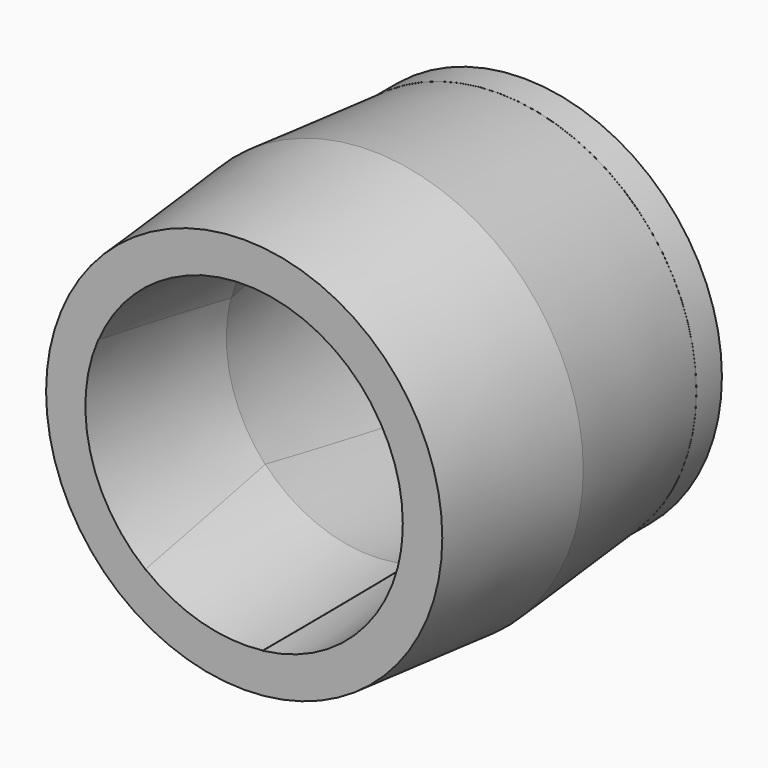
from build123d import *

# Parameters (mm, degrees)
F0_R                   = 31.1969558242
F0_R_2                 = 5
F1_DEPTH               = 5
F2_R                   = 31.1829801171
F3_DEPTH               = 25
DRAFT_F3_DRAFTED_ANGLE = -5
F4_DEPTH               = 25
DRAFT_F4_DRAFTED_ANGLE = 5


# Not quite as in the source:
# - an extrude with a draft is written as a straight extrude whose walls are then drafted


with BuildPart() as f1:
    # F0 (on Front) → F1 (new body)
    with BuildSketch(Plane.XZ):
        with Locations((-39.6958890117, 37.1901692524)):
            Circle(F0_R)
        with BuildLine():
            ThreePointArc((-55.2495512535, 17.6176479313), (-63.9407116305, 31.091925556), (-62.6588155755, 47.0747028086))
            Line((-62.6588155755, 47.0747028086), (-50.450664133, 34.4850457453))
            Line((-50.450664133, 34.4850457453), (-55.2495512535, 17.6176479313))
        make_face(mode=Mode.SUBTRACT)
        with BuildLine():
            Line((-36.774682894, 12.3614247248), (-31.9757957735, 29.2288225388))
            Line((-31.9757957735, 29.2288225388), (-14.9687572105, 33.5065632896))
            ThreePointArc((-14.9687572105, 33.5065632896), (-22.2922437427, 19.2426588025), (-36.774682894, 12.3614247248))
        make_face(mode=Mode.SUBTRACT)
        with Locations((-39.6958890117, 37.1901692524)):
            Circle(F0_R_2, mode=Mode.SUBTRACT)
        with BuildLine():
            ThreePointArc((-48.8693585709, 60.4462965363), (-32.8547116618, 61.2359233988), (-19.6541685655, 52.1343802238))
            Line((-19.6541685655, 52.1343802238), (-36.6612071285, 47.856639473))
            Line((-36.6612071285, 47.856639473), (-48.8693585709, 60.4462965363))
        make_face(mode=Mode.SUBTRACT)
    extrude(amount=F1_DEPTH)


with BuildPart() as f3_drafted:
    # F2 (on face) → F3 (new body)
    with BuildSketch(Plane.XZ.offset(5)):
        with Locations((-39.6958890117, 37.1901692524)):
            Circle(F2_R)
        with BuildLine():
            ThreePointArc((-19.6928828109, 52.1246425199), (-16.0052078333, 45.0584838212), (-14.7327411964, 37.1901692524))
            ThreePointArc((-14.7327411964, 37.1901692524), (-14.8015185073, 35.3383954976), (-15.0074714559, 33.4968255857))
            Line((-15.0074714559, 33.4968255857), (-14.9687572105, 33.5065632896))
            ThreePointArc((-14.9687572105, 33.5065632896), (-22.2922437427, 19.2426588025), (-36.774682894, 12.3614247248))
            Line((-36.774682894, 12.3614247248), (-36.7637588703, 12.3998210967))
            ThreePointArc((-36.7637588703, 12.3998210967), (-46.5269818682, 13.179860649), (-55.2386272298, 17.6560443032))
            Line((-55.2386272298, 17.6560443032), (-55.2495512535, 17.6176479313))
            ThreePointArc((-55.2495512535, 17.6176479313), (-63.9407116305, 31.091925556), (-62.6588155755, 47.0747028086))
            Line((-62.6588155755, 47.0747028086), (-62.6310253539, 47.0460441406))
            ThreePointArc((-62.6310253539, 47.0460441406), (-57.0738797867, 55.1112235035), (-48.8415683493, 60.4176378682))
            Line((-48.8415683493, 60.4176378682), (-48.8693585709, 60.4462965363))
            ThreePointArc((-48.8693585709, 60.4462965363), (-32.8547116618, 61.2359233988), (-19.6541685655, 52.1343802238))
            Line((-19.6541685655, 52.1343802238), (-19.6928828109, 52.1246425199))
        make_face(mode=Mode.SUBTRACT)
    extrude(amount=F3_DEPTH)

    # draft_F3_drafted
    draft_f3_drafted_walls = [f3_drafted.faces().sort_by_distance(p)[0] for p in [
        (-70.8788691288, -21.6666666667, 37.1901692524),
        (-19.6735256882, -21.6666666667, 52.1295113718),
        (-32.8547116618, -21.6666666667, 61.2359233988),
        (-48.8554634601, -21.6666666667, 60.4319672023),
        (-57.0738797867, -21.6666666667, 55.1112235035),
        (-62.6449204647, -21.6666666667, 47.0603734746),
        (-63.9407116305, -21.6666666667, 31.091925556),
        (-55.2440892417, -21.6666666667, 17.6368461172),
        (-46.5269818682, -21.6666666667, 13.179860649),
        (-36.7692208821, -21.6666666667, 12.3806229107),
        (-22.2922437427, -21.6666666667, 19.2426588025),
        (-14.9881143332, -21.6666666667, 33.5016944377),
        (-15.4868053801, -21.6666666667, 43.2794236047),
    ]]
    draft(draft_f3_drafted_walls, neutral_plane=Plane.XZ.offset(5), angle=DRAFT_F3_DRAFTED_ANGLE)


with BuildPart() as f1_1:
    add(f1.part)

    # join_F3_drafted: union F3_drafted
    add(f3_drafted.part)


with BuildPart() as f4_drafted:
    # F4 (new): a face of the model
    f4_faces = [f1_1.part.faces().sort_by_distance(p)[0] for p in [
        (-72.1222340217, -30, 37.1901692524),
    ]]
    extrude(f4_faces, amount=F4_DEPTH)

    # draft_F4_drafted
    draft_f4_drafted_walls = [f4_drafted.faces().sort_by_distance(p)[0] for p in [
        (-73.0660857169, -46.6666666667, 37.1901692524),
        (-17.6079525084, -46.6666666667, 42.7458964138),
        (-17.901251199, -46.6666666667, 30.5136159365),
        (-23.8148654077, -46.6666666667, 20.8128625053),
        (-33.6929425523, -46.6666666667, 15.2004617652),
        (-45.928456405, -46.6666666667, 15.2835915427),
        (-56.3752726993, -46.6666666667, 21.6537358983),
        (-61.8195645022, -46.6666666667, 31.6254527468),
        (-61.741007547, -46.6666666667, 42.9863188646),
        (-55.5512581216, -46.6666666667, 53.5410198006),
        (-44.8111431367, -46.6666666667, 59.4031559224),
        (-33.4532371251, -46.6666666667, 59.132192505),
        (-23.6537169357, -46.6666666667, 53.3837271273),
    ]]
    draft(draft_f4_drafted_walls, neutral_plane=Plane(origin=(-39.6958890117, -30, 37.1901692524), x_dir=(1, 0, 0), z_dir=(0, -1, 0)), angle=DRAFT_F4_DRAFTED_ANGLE)


with BuildPart() as f1_2:
    add(f1_1.part)

    # join_F4_drafted: union F4_drafted
    add(f4_drafted.part)


solid = f1_2.part
